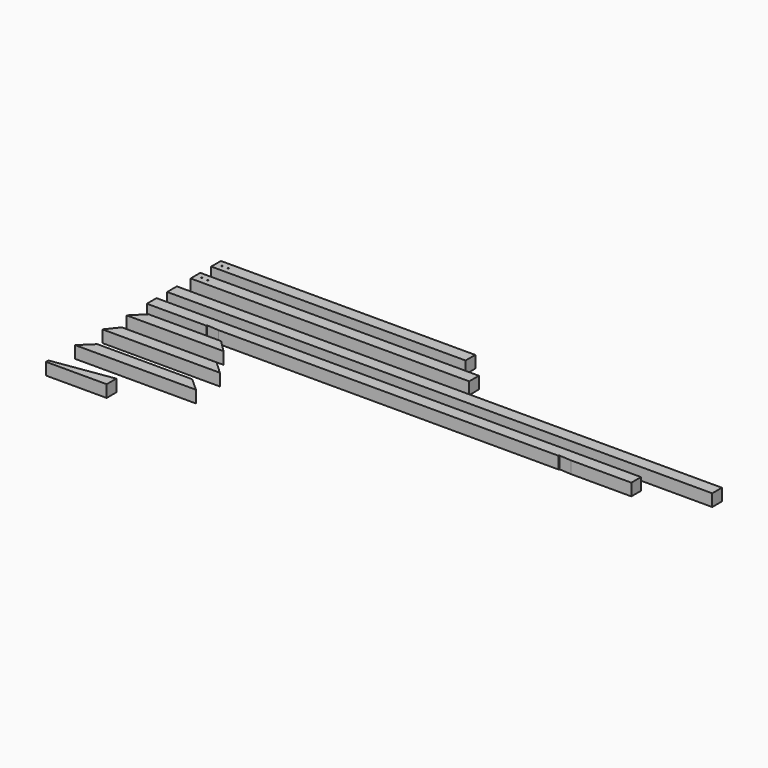
from build123d import *

# Parameters (mm, degrees)
F0_W     = 2100
F0_H     = 100
F0_R     = 5
F1_DEPTH = 100
F0_W_2   = 2300
F0_W_3   = 4500
F0_W_4   = 4000
F2_R     = 5
F3_DEPTH = 50
F5_DEPTH = 100


# Not quite as in the source:
# - a feature names something its author has since deleted; it is built from what else it names


with BuildPart() as f1:
    # F0 (on Top) → F1 (new body)
    with BuildSketch(Plane.XY):
        with Locations((1050, 50)):
            Rectangle(F0_W, F0_H)
        with Locations((50, 50)):
            Circle(F0_R, mode=Mode.SUBTRACT)
        with Locations((100, 50)):
            Circle(F0_R, mode=Mode.SUBTRACT)
    extrude(amount=F1_DEPTH)

    # F2 (on face) → F3 (cut)
    with BuildSketch(Plane(origin=(0, -354.4026255608, 0), x_dir=(-1, 0, 0), z_dir=(0, 1, 0))):
        with Locations((100, 50)):
            Circle(F2_R)
        with Locations((50, 50)):
            Circle(F2_R)
    extrude(amount=-F3_DEPTH, mode=Mode.SUBTRACT)


with BuildPart() as f1b:
    # F0 (on Top) → F1, piece 2 (new body)
    with BuildSketch(Plane.XY):
        with Locations((1150, -162.5102728605)):
            Rectangle(F0_W_2, F0_H)
        with Locations((50, -162.5102728605)):
            Circle(F0_R, mode=Mode.SUBTRACT)
        with Locations((100, -162.5102728605)):
            Circle(F0_R, mode=Mode.SUBTRACT)
    extrude(amount=F1_DEPTH)


with BuildPart() as f1c:
    # F0 (on Top) → F1, piece 3 (new body)
    with BuildSketch(Plane.XY):
        with Locations((2250, -404.4026255608)):
            Rectangle(F0_W_3, F0_H)
    extrude(amount=F1_DEPTH)


with BuildPart() as f1d:
    # F0 (on Top) → F1, piece 4 (new body)
    with BuildSketch(Plane.XY):
        with Locations((2000, -614.3207073212)):
            Rectangle(F0_W_4, F0_H)
    extrude(amount=F1_DEPTH)

    # F4 (on face) → F5 (cut)
    with BuildSketch(Plane.XY.offset(100)):
        Polygon((3500, -664.3207073212), (3400.2363447921, -657.4495284155), (3399.763095296, -664.3207073212), align=None)
        Polygon((492.5, -664.3207073212), (592.736904704, -664.3207073212), (492.9732494961, -657.4495284155), align=None)
    extrude(amount=-F5_DEPTH, mode=Mode.SUBTRACT)


with BuildPart() as f1e:
    # F0 (on Top) → F1, piece 5 (new body)
    with BuildSketch(Plane.XY):
        Polygon((100, -772.8145360947), (0, -872.8145360947), (800, -872.8145360947), (700, -772.8145360947), align=None)
    extrude(amount=F1_DEPTH)


with BuildPart() as f1f:
    # F0 (on Top) → F1, piece 6 (new body)
    with BuildSketch(Plane.XY):
        Polygon((80.9784033195, -1022.974395752), (0, -1122.974395752), (970, -1122.974395752), (862.7631289975, -1022.974395752), align=None)
    extrude(amount=F1_DEPTH)


with BuildPart() as f1g:
    # F0 (on Top) → F1, piece 7 (new body)
    with BuildSketch(Plane.XY):
        Polygon((103.5530313791, -1304.6602249146), (0, -1404.6602249146), (998, -1404.6602249146), (886.9387485171, -1304.6602249146), align=None)
    extrude(amount=F1_DEPTH)


with BuildPart() as f1h:
    # F0 (on Top) → F1, piece 8 (new body)
    with BuildSketch(Plane.XY):
        Polygon((0, -1679.1014432907), (0, -1704.1014432907), (500, -1704.1014432907), (500, -1604.1014432907), align=None)
    extrude(amount=F1_DEPTH)


solid = Compound([f1.part, f1b.part, f1c.part, f1d.part, f1e.part, f1f.part, f1g.part, f1h.part])
